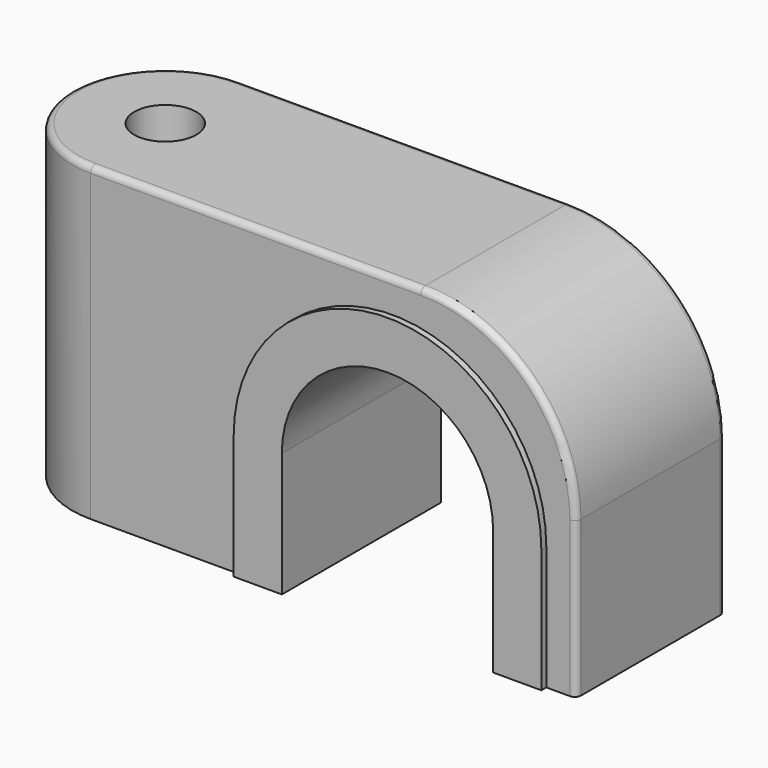
from build123d import *

# Parameters (mm, degrees)
F1_DEPTH      = 3
F2_R          = 1.49999
F4_D          = 1
F5_R          = 2.5
F6_R          = 0.1
F8_DEPTH      = 0.1
F8_DEPTH_BACK = 3.1


# Not quite as in the source:
# - a fillet or chamfer is up to 0.001 mm smaller than in the source, because OpenCascade refuses the exact size


with BuildPart() as f1:
    # F0 (on Front) → F1 (new body)
    with BuildSketch(Plane.XZ):
        with BuildLine():
            Line((0, 5), (0, 0))
            Line((0, 0), (4.6566454311, 0))
            Line((4.6566454311, 0), (4.6566454311, 2))
            ThreePointArc((4.6566454311, 2), (6.3577308128, 3.7010853817), (8.0588161945, 2))
            Line((8.0588161945, 2), (8.0588161945, 0))
            Line((8.0588161945, 0), (9.3132908622, 0))
            Line((9.3132908622, 0), (9.3132908622, 5))
            Line((9.3132908622, 5), (0, 5))
        make_face()
    extrude(amount=F1_DEPTH)

    # F2 (radius 1.5 in the source; OpenCascade refuses exactly that, so slightly less here)
    f2_edges = [f1.edges().sort_by_distance(p)[0] for p in [
        (0, 0, 2.5),
        (0, -3, 2.5),
    ]]
    fillet(f2_edges, radius=F2_R)

    # F4 (through all)
    with Locations(Plane.XY.offset(5)):
        with Locations((1.5, -1.5)):
            Hole(F4_D / 2)

    # F5
    f5_edges = [f1.edges().sort_by_distance(p)[0] for p in [
        (9.313291, -1.5, 5),
    ]]
    fillet(f5_edges, radius=F5_R)

    # F6
    f6_edges = [f1.edges().sort_by_distance(p)[0] for p in [
        (4.15664, -3, 5),
        (8.581058, -3, 4.267767),
        (9.313291, -3, 1.25),
        (9.313291, 0, 1.25),
        (8.581058, 0, 4.267767),
        (4.15664, 0, 5),
    ]]
    fillet(f6_edges, radius=F6_R)

    # F7 (on face) → F8 (join, two sides)
    with BuildSketch(Plane.XZ.offset(3)) as f8_sk:
        with BuildLine():
            Line((3.8816455076, 2), (3.8816455076, 0))
            Line((3.8816455076, 0), (4.6566454311, 0))
            Line((4.6566454311, 0), (4.6566454311, 2))
            ThreePointArc((4.6566454311, 2), (6.3577308128, 3.7010853817), (8.0588161945, 2))
            Line((8.0588161945, 2), (8.0588161945, 0))
            Line((8.0588161945, 0), (8.833816118, 0))
            Line((8.833816118, 0), (8.833816118, 2))
            ThreePointArc((8.833816118, 2), (6.3577308128, 4.4760853052), (3.8816455076, 2))
        make_face()
    extrude(amount=F8_DEPTH)
    extrude(f8_sk.sketch, amount=-F8_DEPTH_BACK)


solid = f1.part
